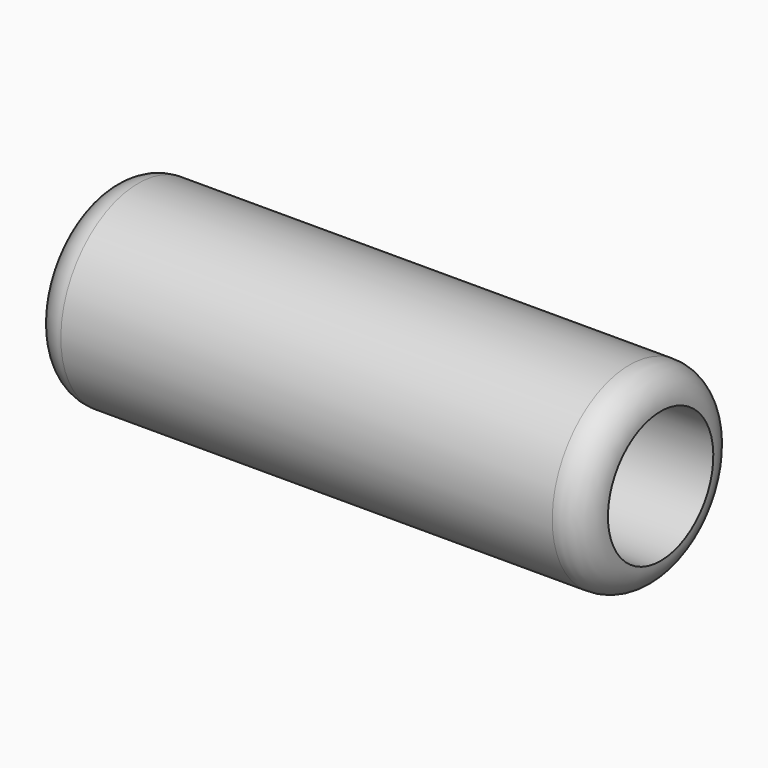
from build123d import *

# Parameters (mm, degrees)
F2_R = 6.34999


# Not quite as in the source:
# - a fillet or chamfer is up to 0.001 mm smaller than in the source, because OpenCascade refuses the exact size


with BuildPart() as f1:
    # F0 (on Front) → F1 (revolve)
    with BuildSketch(Plane.XZ):
        Polygon((3.9624, -5.7219677535), (0, -5.7219677535), (0, -23.1971677535), (113.5126, -23.1971677535), (113.5126, -16.8471677535), (3.9624, -16.8471677535), align=None)
    revolve(axis=Axis((1.9812, 0, -3.3343677535), (1, 0, 0)))

    # F2 (radius 6.35 in the source; OpenCascade refuses exactly that, so slightly less here)
    f2_edges = [f1.edges().sort_by_distance(p)[0] for p in [
        (0, 0, 16.528432),
        (113.5126, 0, 16.528432),
    ]]
    fillet(f2_edges, radius=F2_R)


solid = f1.part
